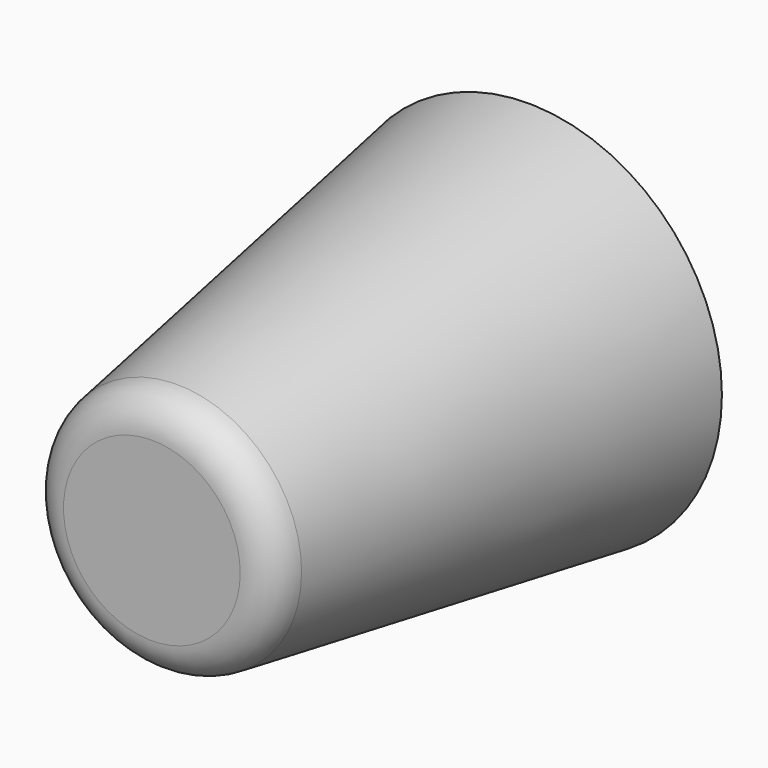
from build123d import *

# Parameters (mm, degrees)
F0_R     = 12
F1_DEPTH = 25.5
F3_R     = 2
F4_R     = 8.25
F5_DEPTH = 2
F6_R     = 1.5
F7_DEPTH = 20


# Not quite as in the source:
# - a fillet or chamfer that OpenCascade refuses, or shapes differently, is made with other operations: its cross-section is extruded or revolved along the edge and cut away or added


with BuildPart() as f1:
    # F0 (on Front) → F1 (new body)
    with BuildSketch(Plane.XZ):
        Circle(F0_R)
    extrude(amount=F1_DEPTH)

    # F2: chamfer of 5.5 x 35 on 1 edges, made by hand

    # F2_s1 → F2_t2 (revolve, cut)
    with BuildSketch(Plane.XY):
        Polygon((12, 9.5), (6.5, -25.5), (12, -25.5), align=None)
    revolve(axis=Axis((0, -25.5, 0), (0, -1, 0)), mode=Mode.SUBTRACT)

    # F3
    f3_edges = [f1.edges().sort_by_distance(p)[0] for p in [
        (-6.5, -25.5, 0),
    ]]
    fillet(f3_edges, radius=F3_R)

    # F4 (on face) → F5 (join)
    with BuildSketch(Plane(origin=(0, 0, 0), x_dir=(-1, 0, 0), z_dir=(0, 1, 0))):
        Circle(F4_R)
    extrude(amount=F5_DEPTH)

    # F6 (on face) → F7 (cut)
    with BuildSketch(Plane(origin=(0, 2, 0), x_dir=(-1, 0, 0), z_dir=(0, 1, 0))):
        Circle(F6_R)
    extrude(amount=-F7_DEPTH, mode=Mode.SUBTRACT)


solid = f1.part
